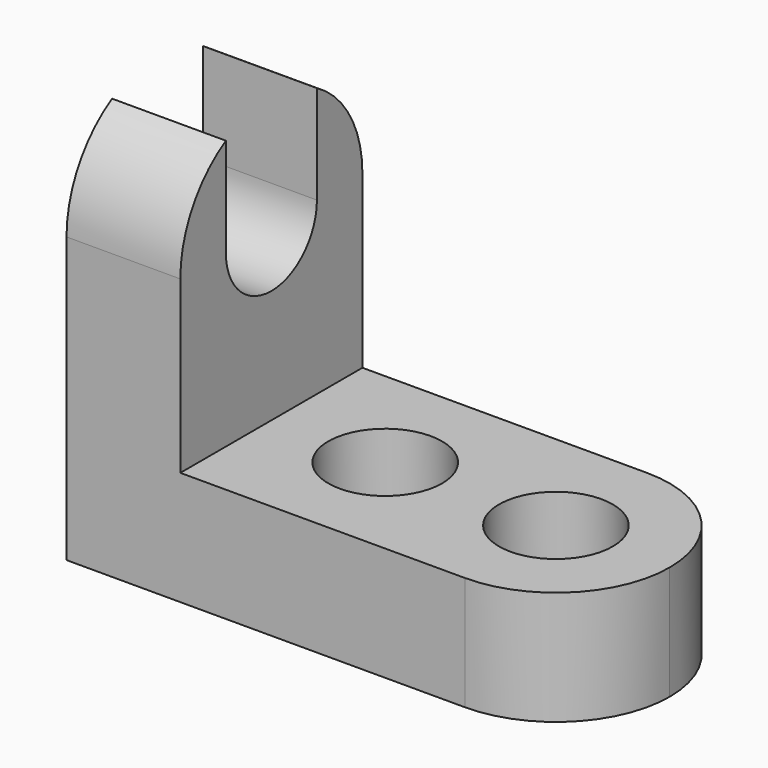
from build123d import *

# Parameters (mm, degrees)
F1_DEPTH  = 25.4
F3_DEPTH  = 25.4
F5_DEPTH  = 25.4
F6_R      = 6.35
F7_DEPTH  = 25.4
F9_DEPTH  = 25.4
F11_DEPTH = 25.4


with BuildPart() as f1:
    # F0 (on Front) → F1 (new body)
    with BuildSketch(Plane.XZ):
        Polygon((-53.4433176321, 48.6006695512), (-66.1433176321, 48.6006695512), (-66.1433176321, -2.1993304488), (-8.9933176321, -2.1993304488), (-8.9933176321, 10.5006695512), (-53.4433176321, 10.5006695512), align=None)
    extrude(amount=F1_DEPTH)

    # F2 (on face) → F3 (cut)
    with BuildSketch(Plane.YZ.offset(-53.4433176321)):
        with BuildLine():
            ThreePointArc((-25.4, 35.9006695512), (-21.6802561211, 44.8809256722), (-12.7, 48.6006695512))
            Line((-12.7, 48.6006695512), (-25.4, 48.6006695512))
            Line((-25.4, 48.6006695512), (-25.4, 35.9006695512))
        make_face()
        with BuildLine():
            ThreePointArc((-12.7, 48.6006695512), (-3.7197438789, 44.8809256722), (0, 35.9006695512))
            Line((0, 35.9006695512), (0, 48.6006695512))
            Line((0, 48.6006695512), (-12.7, 48.6006695512))
        make_face()
    extrude(amount=-F3_DEPTH, mode=Mode.SUBTRACT)

    # F4 (on face) → F5 (cut)
    with BuildSketch(Plane.YZ.offset(-53.4433176321)):
        with BuildLine():
            Line((-19.05, 46.8991921792), (-19.05, 29.5506688558))
            ThreePointArc((-19.05, 29.5506688558), (-12.6999996523, 23.2006695512), (-6.35, 29.5506695512))
            Line((-6.35, 29.5506695512), (-6.35, 46.8991921792))
            ThreePointArc((-6.35, 46.8991921792), (-12.7, 48.6006695512), (-19.05, 46.8991921792))
        make_face()
    extrude(amount=-F5_DEPTH, mode=Mode.SUBTRACT)

    # F6 (on face) → F7 (cut)
    with BuildSketch(Plane.XY.offset(10.5006695512)):
        with Locations((-21.6933176321, -12.7)):
            Circle(F6_R)
        with Locations((-40.7433176321, -12.7)):
            Circle(F6_R)
    extrude(amount=-F7_DEPTH, mode=Mode.SUBTRACT)

    # F8 (on face) → F9 (cut)
    with BuildSketch(Plane.XY.offset(10.5006695512)):
        with BuildLine():
            ThreePointArc((-21.6933176321, 0), (-12.713061511, -3.7197438789), (-8.9933176321, -12.7))
            Line((-8.9933176321, -12.7), (-8.9933176321, 0))
            Line((-8.9933176321, 0), (-21.6933176321, 0))
        make_face()
        with BuildLine():
            ThreePointArc((-8.9933176321, -12.7), (-12.713061511, -21.6802561211), (-21.6933176321, -25.4))
            Line((-21.6933176321, -25.4), (-8.9933176321, -25.4))
            Line((-8.9933176321, -25.4), (-8.9933176321, -12.7))
        make_face()
    extrude(amount=-F9_DEPTH, mode=Mode.SUBTRACT)

    # F10 (on face) → F11 (cut)
    with BuildSketch(Plane.YZ.offset(-53.4433176321)):
        with BuildLine():
            ThreePointArc((-25.4, 29.5506695512), (-23.6985226281, 35.9006695512), (-19.05, 40.5491921792))
            Line((-19.05, 40.5491921792), (-19.05, 46.8991921792))
            ThreePointArc((-19.05, 46.8991921792), (-23.6985226281, 42.2506695512), (-25.4, 35.9006695512))
            Line((-25.4, 35.9006695512), (-25.4, 29.5506695512))
        make_face()
        with BuildLine():
            ThreePointArc((-6.35, 40.5491921792), (-1.7014773719, 35.9006695512), (0, 29.5506695512))
            Line((0, 29.5506695512), (0, 35.9006695512))
            ThreePointArc((0, 35.9006695512), (-1.7014773719, 42.2506695512), (-6.35, 46.8991921792))
            Line((-6.35, 46.8991921792), (-6.35, 40.5491921792))
        make_face()
    extrude(amount=-F11_DEPTH, mode=Mode.SUBTRACT)


solid = f1.part
